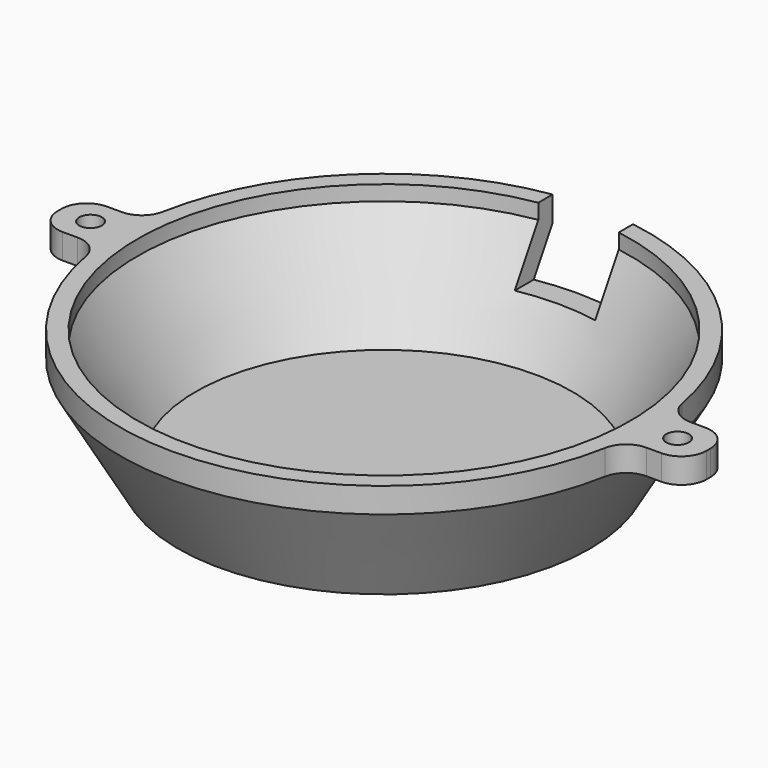
from build123d import *

# Parameters (mm, degrees)
F0_R        = 52.5
F0_R_2      = 49
F1_DEPTH    = 2
F2_DEPTH    = 25
F3_SIZE2    = 11.5470053838
F3_SIZE     = 20
F4_SIZE2    = 11.5470053838
F4_SIZE     = 20
F6_DEPTH    = 13
F7_R        = 2.25
F8_DEPTH    = 5
F9_T1_DEPTH = 5
F9_T3_DEPTH = 5


# Not quite as in the source:
# - a fillet or chamfer that OpenCascade refuses, or shapes differently, is made with other operations: its cross-section is extruded or revolved along the edge and cut away or added


with BuildPart() as f1:
    # F0 (on Top) → F1 (new body)
    with BuildSketch(Plane.XY):
        Circle(F0_R)
        Circle(F0_R_2, mode=Mode.SUBTRACT)
        Circle(F0_R_2)
    extrude(amount=F1_DEPTH)

    # F0 (on Top) → F2 (join)
    with BuildSketch(Plane.XY):
        Circle(F0_R)
        Circle(F0_R_2, mode=Mode.SUBTRACT)
    extrude(amount=F2_DEPTH)

    # F3
    f3_edges = [f1.edges().sort_by_distance(p)[0] for p in [
        (-49, 0, 2),
    ]]
    chamfer(f3_edges, length=F3_SIZE, length2=F3_SIZE2)

    # F4
    f4_edges = [f1.edges().sort_by_distance(p)[0] for p in [
        (-52.5, 0, 0),
    ]]
    f4_side = f1.faces().sort_by_distance((-52.5, 0, 12.5))[0]
    chamfer(f4_edges, length=F4_SIZE, length2=F4_SIZE2, reference=f4_side)

    # F5 (on face) → F6 (cut)
    with BuildSketch(Plane.XY.offset(25)):
        with BuildLine():
            Line((8, 51.8868962263), (8, 67.5))
            Line((8, 67.5), (-8, 67.5))
            Line((-8, 67.5), (-8, 51.8868962263))
            ThreePointArc((-8, 51.8868962263), (0, 52.5), (8, 51.8868962263))
        make_face()
        with BuildLine():
            Line((8, 48.3425278611), (8, 51.8868962263))
            ThreePointArc((8, 51.8868962263), (0, 52.5), (-8, 51.8868962263))
            Line((-8, 51.8868962263), (-8, 48.3425278611))
            ThreePointArc((-8, 48.3425278611), (0, 49), (8, 48.3425278611))
        make_face()
        with BuildLine():
            Line((8, 37.5), (8, 48.3425278611))
            ThreePointArc((8, 48.3425278611), (0, 49), (-8, 48.3425278611))
            Line((-8, 48.3425278611), (-8, 37.5))
            Line((-8, 37.5), (8, 37.5))
        make_face()
    extrude(amount=-F6_DEPTH, mode=Mode.SUBTRACT)

    # F7 (on face) → F8 (join)
    with BuildSketch(Plane.XY.offset(25)):
        with BuildLine():
            Line((-64.5158270159, -5.4877443216), (-52.2123995068, -5.4877443216))
            ThreePointArc((-52.2123995068, -5.4877443216), (-52.5, 0), (-52.2123995068, 5.4877443216))
            Line((-52.2123995068, 5.4877443216), (-64.5158270159, 5.4877443216))
            Line((-64.5158270159, 5.4877443216), (-64.5158270159, -5.4877443216))
        make_face()
        with Locations((-58.3641132614, 0)):
            Circle(F7_R, mode=Mode.SUBTRACT)
        with BuildLine():
            ThreePointArc((52.2123995068, 5.4877443216), (52.5, 0), (52.2123995068, -5.4877443216))
            Line((52.2123995068, -5.4877443216), (64.5158270159, -5.4877443216))
            Line((64.5158270159, -5.4877443216), (64.5158270159, 5.4877443216))
            Line((64.5158270159, 5.4877443216), (52.2123995068, 5.4877443216))
        make_face()
        with Locations((58.3641132614, 0)):
            Circle(F7_R, mode=Mode.SUBTRACT)
    extrude(amount=-F8_DEPTH)

    # F9: fillet of radius 5 on 8 edges, made by hand

    # F9_s2 → F9_t1 (join)
    with BuildSketch(Plane.XY.offset(20)):
        with BuildLine():
            ThreePointArc((-51.6193248202, -9.5757665545), (-53.3385688277, -6.6432749931), (-56.5354509936, -5.4877443216))
            Line((-56.5354509936, -5.4877443216), (-56.5354509936, -5.3877443216))
            Line((-56.5354509936, -5.3877443216), (-52.2123995068, -5.3877443216))
            Line((-52.2123995068, -5.3877443216), (-52.1129473173, -5.4772914752))
            ThreePointArc((-52.1129473173, -5.4772914752), (-51.8571206165, -7.5232334382), (-51.5210022967, -9.5575269991))
            Line((-51.5210022967, -9.5575269991), (-51.6193248202, -9.5757665545))
        make_face()
        with BuildLine():
            ThreePointArc((-51.6193248202, 9.5757665545), (-53.3385688277, 6.6432749931), (-56.5354509936, 5.4877443216))
            Line((-56.5354509936, 5.4877443216), (-56.5354509936, 5.3877443216))
            Line((-56.5354509936, 5.3877443216), (-52.2123995068, 5.3877443216))
            Line((-52.2123995068, 5.3877443216), (-52.1129473173, 5.4772914752))
            ThreePointArc((-52.1129473173, 5.4772914752), (-51.8571206165, 7.5232334382), (-51.5210022967, 9.5575269991))
            Line((-51.5210022967, 9.5575269991), (-51.6193248202, 9.5757665545))
        make_face()
        with BuildLine():
            ThreePointArc((51.6193248202, -9.5757665545), (53.3385688277, -6.6432749931), (56.5354509936, -5.4877443216))
            Line((56.5354509936, -5.4877443216), (56.5354509936, -5.3877443216))
            Line((56.5354509936, -5.3877443216), (52.2123995068, -5.3877443216))
            Line((52.2123995068, -5.3877443216), (52.1129473173, -5.4772914752))
            ThreePointArc((52.1129473173, -5.4772914752), (51.8571206165, -7.5232334382), (51.5210022967, -9.5575269991))
            Line((51.5210022967, -9.5575269991), (51.6193248202, -9.5757665545))
        make_face()
        with BuildLine():
            ThreePointArc((51.6193248202, 9.5757665545), (53.3385688277, 6.6432749931), (56.5354509936, 5.4877443216))
            Line((56.5354509936, 5.4877443216), (56.5354509936, 5.3877443216))
            Line((56.5354509936, 5.3877443216), (52.2123995068, 5.3877443216))
            Line((52.2123995068, 5.3877443216), (52.1129473173, 5.4772914752))
            ThreePointArc((52.1129473173, 5.4772914752), (51.8571206165, 7.5232334382), (51.5210022967, 9.5575269991))
            Line((51.5210022967, 9.5575269991), (51.6193248202, 9.5757665545))
        make_face()
    extrude(amount=F9_T1_DEPTH)

    # F9_s4 → F9_t3 (cut)
    with BuildSketch(Plane.XY.offset(20)):
        with BuildLine():
            ThreePointArc((-59.5158270159, -5.4877443216), (-63.0513609218, -4.0232782275), (-64.5158270159, -0.4877443216))
            Line((-64.5158270159, -0.4877443216), (-64.6158270159, -0.4877443216))
            Line((-64.6158270159, -0.4877443216), (-64.6158270159, -5.5877443216))
            Line((-64.6158270159, -5.5877443216), (-59.5158270159, -5.5877443216))
            Line((-59.5158270159, -5.5877443216), (-59.5158270159, -5.4877443216))
        make_face()
        with BuildLine():
            ThreePointArc((-64.5158270159, 0.4877443216), (-63.0513609218, 4.0232782275), (-59.5158270159, 5.4877443216))
            Line((-59.5158270159, 5.4877443216), (-59.5158270159, 5.5877443216))
            Line((-59.5158270159, 5.5877443216), (-64.6158270159, 5.5877443216))
            Line((-64.6158270159, 5.5877443216), (-64.6158270159, 0.4877443216))
            Line((-64.6158270159, 0.4877443216), (-64.5158270159, 0.4877443216))
        make_face()
        with BuildLine():
            ThreePointArc((64.5158270159, -0.4877443216), (63.0513609218, -4.0232782275), (59.5158270159, -5.4877443216))
            Line((59.5158270159, -5.4877443216), (59.5158270159, -5.5877443216))
            Line((59.5158270159, -5.5877443216), (64.6158270159, -5.5877443216))
            Line((64.6158270159, -5.5877443216), (64.6158270159, -0.4877443216))
            Line((64.6158270159, -0.4877443216), (64.5158270159, -0.4877443216))
        make_face()
        with BuildLine():
            ThreePointArc((59.5158270159, 5.4877443216), (63.0513609218, 4.0232782275), (64.5158270159, 0.4877443216))
            Line((64.5158270159, 0.4877443216), (64.6158270159, 0.4877443216))
            Line((64.6158270159, 0.4877443216), (64.6158270159, 5.5877443216))
            Line((64.6158270159, 5.5877443216), (59.5158270159, 5.5877443216))
            Line((59.5158270159, 5.5877443216), (59.5158270159, 5.4877443216))
        make_face()
    extrude(amount=F9_T3_DEPTH, mode=Mode.SUBTRACT)


solid = f1.part
